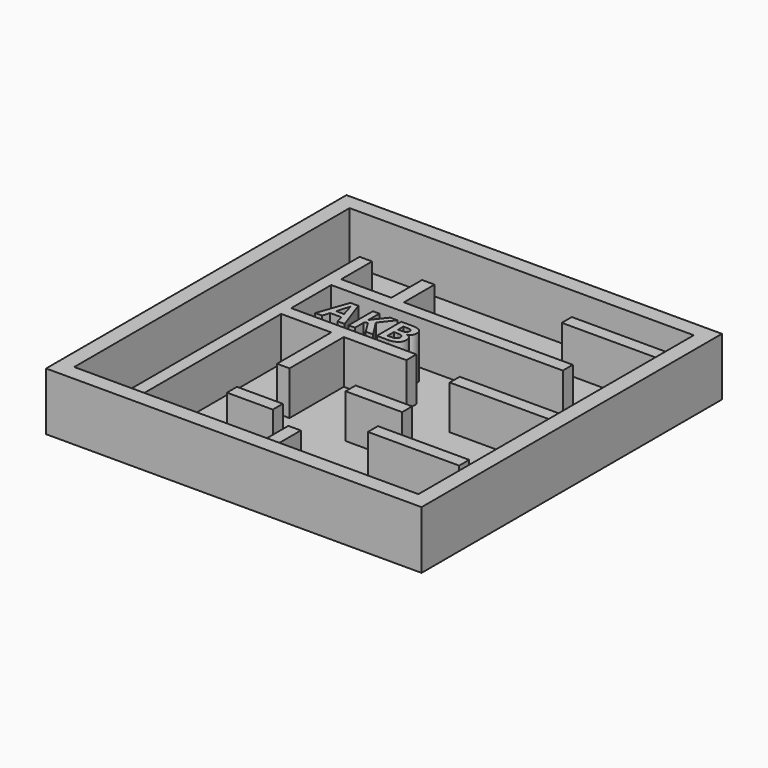
from build123d import *

# Parameters (mm, degrees)
F0_W         = 38.1
F0_H         = 38.1
F1_DEPTH     = 0.79375
F2_W         = 38.1
F2_H         = 38.1
F2_W_2       = 34.925
F2_H_2       = 34.925
F3_DEPTH     = 5.08
F4_W         = 5.7372341398
F4_H         = 1.27
F4_W_2       = 4.6556494695
F4_W_3       = 1.27
F4_H_2       = 3.6643798614
F4_W_4       = 9.2615359463
F4_W_5       = 10.795
F4_W_6       = 10.2603184734
F5_DEPTH     = 4.445
F6_R         = 1.27
F7_DEPTH     = 0.396875
F8_DEPTH     = 0.396875
F9_TEXT_SIZE = 4.33167378
F10_DEPTH    = 4.445


# Not quite as in the source:
# - Text() gives the source's letters only with a copy of the font that has no kerning and outlines rounded to 1/6400 em; it was checked with that copy


with BuildPart() as f1:
    # F0 (on Top) → F1 (new body)
    with BuildSketch(Plane.XY):
        with Locations((-2.5349948555, 3.3342581889)):
            Rectangle(F0_W, F0_H)
    extrude(amount=F1_DEPTH)

    # F2 (on face) → F3 (join)
    with BuildSketch(Plane.XY.offset(0.79375)):
        with Locations((-2.5349948555, 3.3342581889)):
            Rectangle(F2_W, F2_H)
        with Locations((-2.5349948555, 3.3342581889)):
            Rectangle(F2_W_2, F2_H_2, mode=Mode.SUBTRACT)
    extrude(amount=F3_DEPTH)

    # F4 (on face) → F5 (join)
    with BuildSketch(Plane.XY.offset(0.79375)):
        Polygon((-14.9174948555, 15.7167581889), (-14.9174948555, -14.1282418111), (-13.6474948555, -14.1282418111), (-13.6474948555, 4.1831223458), (-13.6474948555, 5.4531223458), (-13.6474948555, 10.5331223458), (-13.6474948555, 11.8031223458), (-13.6474948555, 15.7167581889), align=None)
        Polygon((-13.6474948555, 5.4531223458), (-13.6474948555, 4.1831223458), (-8.5674948555, 4.1831223458), (-8.5674948555, -2.6982418111), (-7.2974948555, -2.6982418111), (-7.2974948555, 4.1831223458), (-0.9474948555, 4.1831223458), (-0.9474948555, 5.4531223458), align=None)
        Polygon((-8.5674948555, 11.8031223458), (-13.6474948555, 11.8031223458), (-13.6474948555, 10.5331223458), (9.8475051445, 10.5331223458), (9.8475051445, 11.8031223458), (-7.2974948555, 11.8031223458), (-7.2974948555, 15.7038011742), (-8.5674948555, 15.7038011742), align=None)
        with Locations((1.4975465601, -2.3553582763)):
            Rectangle(F4_W, F4_H)
        with Locations((-6.2396701208, -8.4132418111)):
            Rectangle(F4_W_2, F4_H)
        with Locations((-0.5721494712, -12.2960518804)):
            Rectangle(F4_W_3, F4_H_2)
        with Locations((8.9969316032, -6.699264461)):
            Rectangle(F4_W_4, F4_H)
        with Locations((9.5300051445, 3.9692581889)):
            Rectangle(F4_W_5, F4_H)
        with Locations((9.7973459078, 17.5181223458)):
            Rectangle(F4_W_6, F4_H)
    extrude(amount=F5_DEPTH)

    # F6 (on face) → F7 (cut)
    with BuildSketch(Plane.XY.offset(0.79375)):
        with Locations((-17.5219778903, -11.0068349168)):
            Circle(F6_R)
        with Locations((10.1926291827, -11.2294591963)):
            Circle(F6_R)
    extrude(amount=-F7_DEPTH, mode=Mode.SUBTRACT)

    # F6 (on face) → F8 (cut)
    with BuildSketch(Plane.XY.offset(0.79375)):
        with Locations((-17.5219778903, -11.0068349168)):
            Circle(F6_R)
        with Locations((10.1926291827, -11.2294591963)):
            Circle(F6_R)
    extrude(amount=-F8_DEPTH, mode=Mode.SUBTRACT)

    # F9 (on face) → F10 (join)
    with BuildSketch(Plane.XY.offset(0.79375)):
        with Locations((-11.6382306442, 5.9887734242)):
            Text('AKB', F9_TEXT_SIZE, font='Open Sans', font_style=FontStyle.BOLD, text_align=(TextAlign.LEFT, TextAlign.BOTTOM))
    extrude(amount=F10_DEPTH)


solid = f1.part
